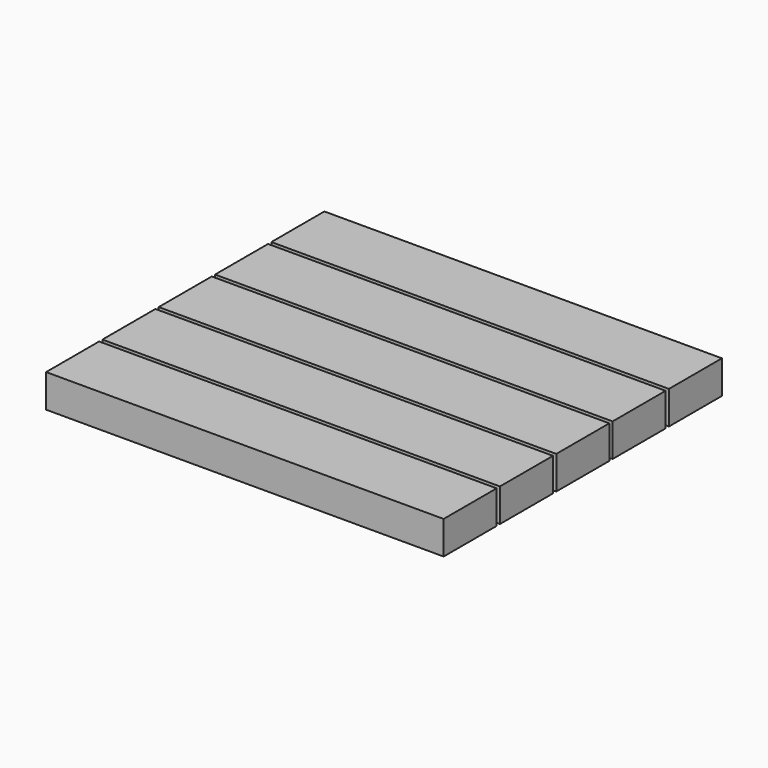
from build123d import *

# Parameters (mm, degrees)
F0_W      = 304.8
F0_H      = 50.8
F1_DEPTH  = 25.4
F2_W      = 304.8
F2_H      = 50.8
F1_FACE_W = 304.8
F1_FACE_H = 50.8
F3_DEPTH  = 25.4


with BuildPart() as f1:
    # F0 (on Top) → F1 (new body)
    with BuildSketch(Plane.XY):
        with Locations((152.4, 25.4)):
            Rectangle(F0_W, F0_H)
    extrude(amount=F1_DEPTH)

    # F2 (on face) + F1_face (on face) → F3 (cut)
    with BuildSketch(Plane.XY.offset(25.4)):
        with Locations((152.4, 25.4)):
            Rectangle(F2_W, F2_H)
    with BuildSketch(Plane(origin=(152.4, 25.4, 25.4), x_dir=(1, 0, 0), z_dir=(0, 0, 1))):
        with Locations((0, -53.975)):
            Rectangle(F1_FACE_W, F1_FACE_H)
    extrude(amount=-F3_DEPTH, mode=Mode.SUBTRACT)


with BuildPart() as f1b:
    # F0 (on Top) → F1, piece 2 (new body)
    with BuildSketch(Plane.XY):
        with Locations((152.4, -28.575)):
            Rectangle(F0_W, F0_H)
    extrude(amount=F1_DEPTH)


with BuildPart() as f1c:
    # F0 (on Top) → F1, piece 3 (new body)
    with BuildSketch(Plane.XY):
        with Locations((152.4, -82.55)):
            Rectangle(F0_W, F0_H)
    extrude(amount=F1_DEPTH)


with BuildPart() as f1d:
    # F0 (on Top) → F1, piece 4 (new body)
    with BuildSketch(Plane.XY):
        with Locations((152.4, -136.525)):
            Rectangle(F0_W, F0_H)
    extrude(amount=F1_DEPTH)


with BuildPart() as f1e:
    # F0 (on Top) → F1, piece 5 (new body)
    with BuildSketch(Plane.XY):
        with Locations((152.4, -190.5)):
            Rectangle(F0_W, F0_H)
    extrude(amount=F1_DEPTH)


with BuildPart() as f1f:
    # F0 (on Top) → F1, piece 6 (new body)
    with BuildSketch(Plane.XY):
        with Locations((152.4, -244.475)):
            Rectangle(F0_W, F0_H)
    extrude(amount=F1_DEPTH)


solid = Compound([f1b.part, f1c.part, f1d.part, f1e.part, f1f.part])
